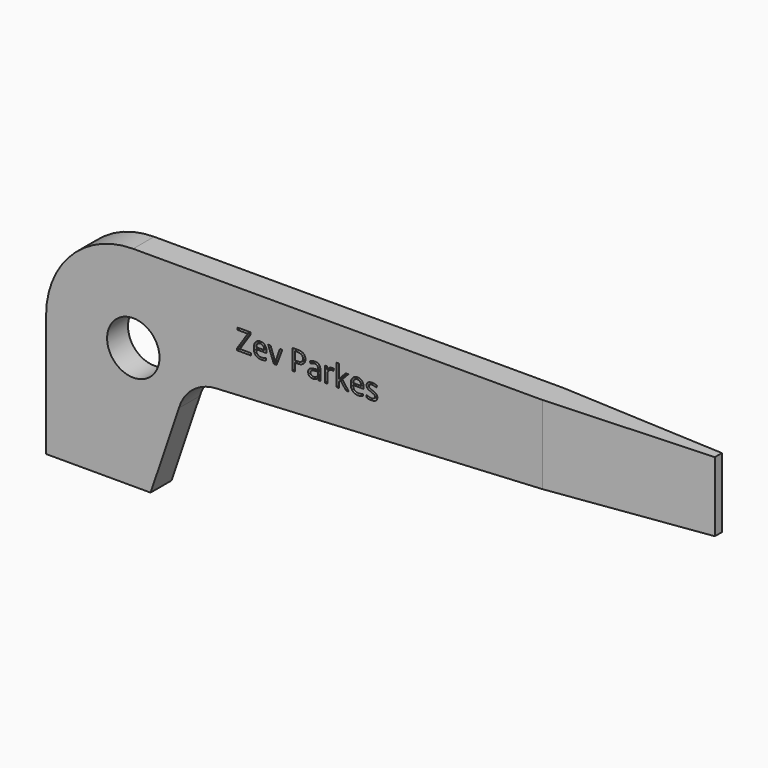
from build123d import *

# Parameters (mm, degrees)
F1_DEPTH     = 2.38125
F2_R         = 2.3876
F3_DEPTH     = 25.4
F5_DEPTH     = 25.4
F6_TEXT_SIZE = 2.5904426972
F7_DEPTH     = 0.508


# Not quite as in the source:
# - a length typed as a fraction of an inch, garbled in the dataset ("3 / 203.2 mm" for 3/8 in), is restored
# - Text() gives the source's letters only with a copy of the font that has no kerning and outlines rounded to 1/6400 em; it was checked with that copy


with BuildPart() as f1:
    # F0 (on Front) → F1 (new body)
    with BuildSketch(Plane.XZ):
        with BuildLine():
            Line((60.325, 19.05), (7.9375, 19.05))
            ThreePointArc((7.9375, 19.05), (2.3248399243, 16.7251600757), (0, 11.1125))
            Line((0, 11.1125), (0, 0))
            Line((0, 0), (9.525, 0))
            Line((9.525, 0), (12.1103451907, 7.6262422093))
            ThreePointArc((12.1103451907, 7.6262422093), (13.3666782674, 9.5039474973), (15.4790089603, 10.3053269279))
            Line((15.4790089603, 10.3053269279), (60.325, 12.7))
            Line((60.325, 12.7), (60.325, 19.05))
        make_face()
    extrude(amount=F1_DEPTH)

    # F2 (on face) → F3 (cut)
    with BuildSketch(Plane.XZ.offset(2.38125)):
        with Locations((7.9502, 11.0998)):
            Circle(F2_R)
    extrude(amount=-F3_DEPTH, mode=Mode.SUBTRACT)

    # F4 (on face) → F5 (cut)
    with BuildSketch(Plane.XY.offset(19.05)):
        Polygon((60.325, -2.38125), (60.325, -1.59385), (45.2374, -2.38125), align=None)
        Polygon((60.325, 0), (45.2374, 0), (60.325, -0.7874), align=None)
    extrude(amount=-F5_DEPTH, mode=Mode.SUBTRACT)

    # F6 (on face) → F7 (cut)
    with BuildSketch(Plane.XZ.offset(2.38125)):
        with Locations((17.3048004508, 13.9776915312)):
            Text('Zev Parkes', F6_TEXT_SIZE, font='Open Sans', text_align=(TextAlign.LEFT, TextAlign.BOTTOM))
    extrude(amount=-F7_DEPTH, mode=Mode.SUBTRACT)


solid = f1.part
